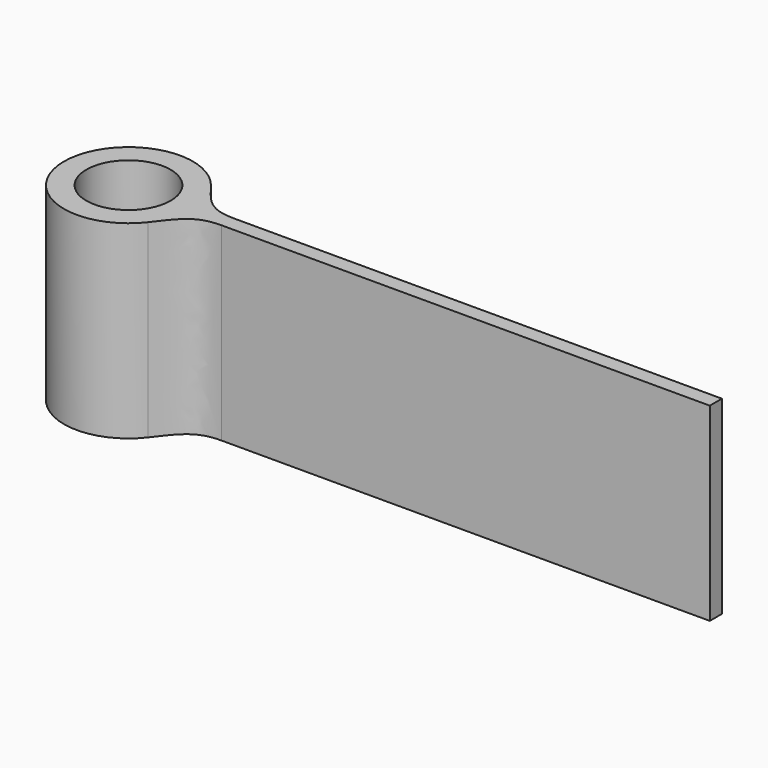
from build123d import *

# Parameters (mm, degrees)
F0_R     = 5.55625
F1_DEPTH = 25


# Not quite as in the source:
# - a feature names something its author has since deleted; it is built from what else it names


with BuildPart() as f1:
    # F0 (on Top) → F1 (new body)
    with BuildSketch(Plane.XY):
        with BuildLine():
            ThreePointArc((-69.0590284919, -1), (-69.0147699554, -0.5008703332), (-69, 0))
            ThreePointArc((-69, 0), (-69.0147699554, 0.5008703332), (-69.0590284919, 1))
            ThreePointArc((-69.0590284919, 1), (-69.6284732517, 3.2076575021), (-70.7642342114, 5.184540408))
            ThreePointArc((-70.7642342114, 5.184540408), (-86, 0), (-70.7642342114, -5.184540408))
            ThreePointArc((-70.7642342114, -5.184540408), (-69.6284732517, -3.2076575021), (-69.0590284919, -1))
        make_face()
        with Locations((-77.5, 0)):
            Circle(F0_R, mode=Mode.SUBTRACT)
        with BuildLine():
            ThreePointArc((-70.7642342114, 5.184540408), (-69.6284732517, 3.2076575021), (-69.0590284919, 1))
            Line((-69.0590284919, 1), (-64.4374042749, 1))
            add(Edge.make_bspline(
                [(-64.4374042749, 1), (-67.7107125521, 1), (-68.7326164375, 2.5450583285), (-70.7642342114, 5.184540408)],
                knots=[0, 0, 0, 0, 7.58545684, 7.58545684, 7.58545684, 7.58545684], degree=3))
        make_face()
        with BuildLine():
            Line((-64.4374042749, -1), (-69.0590284919, -1))
            ThreePointArc((-69.0590284919, -1), (-69.6284732517, -3.2076575021), (-70.7642342114, -5.184540408))
            add(Edge.make_bspline(
                [(-64.4374042749, -1), (-67.7107125521, -1), (-68.7326164375, -2.5450583285), (-70.7642342114, -5.184540408)],
                knots=[0, 0, 0, 0, 7.58545684, 7.58545684, 7.58545684, 7.58545684], degree=3))
        make_face()
        with BuildLine():
            ThreePointArc((-69.0590284919, 1), (-69.0147699554, 0.5008703332), (-69, 0))
            ThreePointArc((-69, 0), (-69.0147699554, -0.5008703332), (-69.0590284919, -1))
            Line((-69.0590284919, -1), (-64.4374042749, -1))
            Line((-64.4374042749, -1), (0, -1))
            Line((0, -1), (0, 1))
            Line((0, 1), (-64.4374042749, 1))
            Line((-64.4374042749, 1), (-69.0590284919, 1))
        make_face()
    extrude(amount=F1_DEPTH)


solid = f1.part
